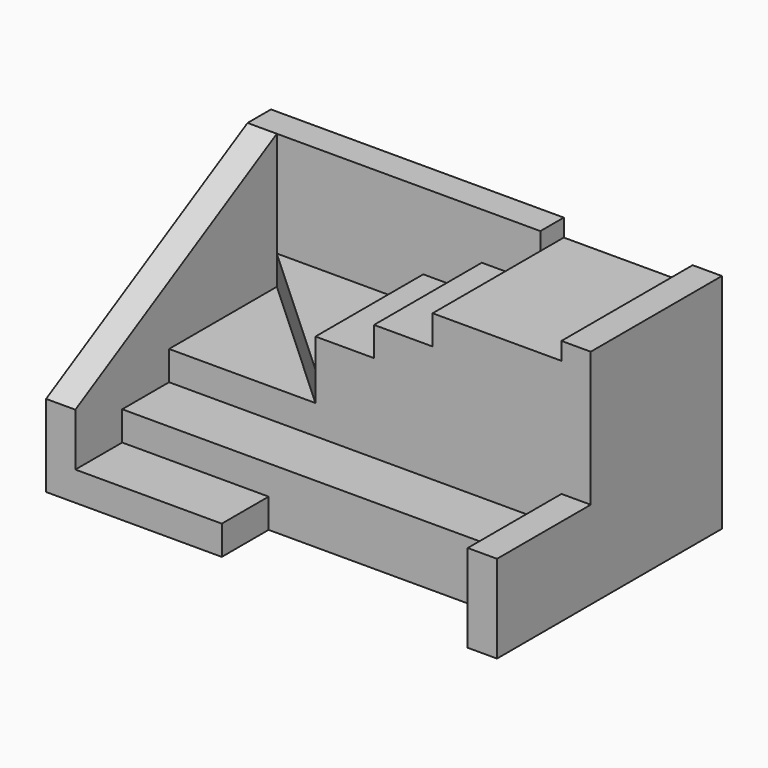
from build123d import *

# Parameters (mm, degrees)
F1_DEPTH  = 38
F0_W      = 25
F0_H      = 10
F3_DEPTH  = 5
F4_DEPTH  = 10
F5_DEPTH  = 15
F6_DEPTH  = 20
F7_DEPTH  = 25
F0_W_2    = 10
F0_H_2    = 23
F8_DEPTH  = 25
F9_DEPTH  = 30
F10_DEPTH = 35
F0_W_3    = 5
F0_H_3    = 28
F11_DEPTH = 38
F12_DEPTH = 15


# Not quite as in the source:
# - a feature names something its author has since deleted; it is built from what else it names


with BuildPart() as f1:
    # F0 (on Top) → F1 (new body)
    with BuildSketch(Plane.XY):
        Polygon((-33.5, 19), (-38.5, 19), (-38.5, -24), (-33.5, -24), (-33.5, -14), (-33.5, -4), align=None)
        Polygon((11.5, 24), (-38.5, 24), (-38.5, 19), (-33.5, 19), (-8.5, 19), (1.5, 19), (11.5, 19), align=None)
    extrude(amount=F1_DEPTH)

    # F0 (on Top) → F3 (join)
    with BuildSketch(Plane.XY):
        with Locations((-21, -19)):
            Rectangle(F0_W, F0_H)
    extrude(amount=F3_DEPTH)

    # F0 (on Top) → F4 (join)
    with BuildSketch(Plane.XY):
        Polygon((33.5, -14), (33.5, -4), (11.5, -4), (1.5, -4), (-8.5, -4), (-33.5, -4), (-33.5, -14), (-8.5, -14), align=None)
    extrude(amount=F4_DEPTH)

    # F0 (on Top) → F5 (join)
    with BuildSketch(Plane.XY):
        Polygon((-8.5, -4), (-33.5, 19), (-33.5, -4), align=None)
    extrude(amount=F5_DEPTH)

    # F0 (on Top) → F6 (join)
    with BuildSketch(Plane.XY):
        Polygon((-8.5, 19), (-33.5, 19), (-8.5, -4), align=None)
    extrude(amount=F6_DEPTH)

    # F2 (on face) → F7 (cut)
    with BuildSketch(Plane.YZ.offset(-33.5)):
        Polygon((-24, 14), (19, 38), (-24, 38), align=None)
    extrude(amount=-F7_DEPTH, mode=Mode.SUBTRACT)

    # F0 (on Top) → F8 (join)
    with BuildSketch(Plane.XY):
        with Locations((-3.5, 7.5)):
            Rectangle(F0_W_2, F0_H_2)
    extrude(amount=F8_DEPTH)

    # F0 (on Top) → F9 (join)
    with BuildSketch(Plane.XY):
        with Locations((6.5, 7.5)):
            Rectangle(F0_W_2, F0_H_2)
    extrude(amount=F9_DEPTH)

    # F0 (on Top) → F10 (join)
    with BuildSketch(Plane.XY):
        Polygon((33.5, 24), (11.5, 24), (11.5, 19), (11.5, -4), (33.5, -4), align=None)
    extrude(amount=F10_DEPTH)

    # F0 (on Top) → F11 (join)
    with BuildSketch(Plane.XY):
        with Locations((36, 10)):
            Rectangle(F0_W_3, F0_H_3)
    extrude(amount=F11_DEPTH)

    # F0 (on Top) → F12 (join)
    with BuildSketch(Plane.XY):
        Polygon((38.5, -4), (33.5, -4), (33.5, -14), (33.5, -24), (38.5, -24), align=None)
    extrude(amount=F12_DEPTH)


solid = f1.part
